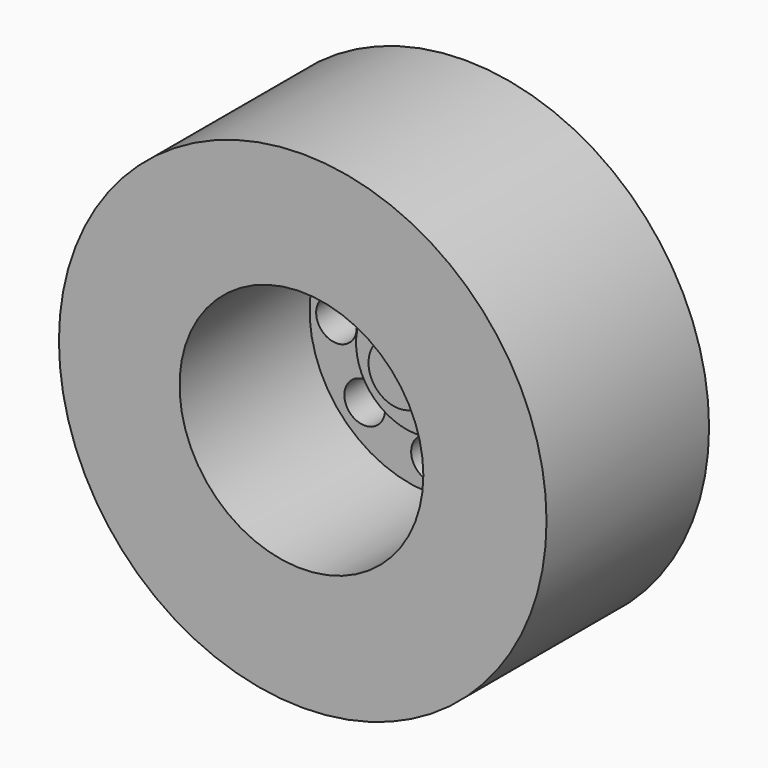
from build123d import *

# Parameters (mm, degrees)
F0_R      = 19.05
F1_DEPTH  = 15.875
F2_R      = 9.525
F3_DEPTH  = 12.7
F4_R      = 1.5875
F5_DEPTH  = 25.4
F6_R      = 1.5875
F7_DEPTH  = 25.4
F8_R      = 1.5875
F9_DEPTH  = 25.4
F10_R     = 1.5875
F11_DEPTH = 25.4
F12_R     = 1.5875
F13_DEPTH = 25.4
F14_R     = 1.5875
F15_DEPTH = 25.4
F16_R     = 1.5875
F17_DEPTH = 25.4
F18_R     = 1.5875
F19_DEPTH = 25.4
F20_R     = 4.7625
F21_DEPTH = 1.5875
F22_R     = 2.38125
F23_DEPTH = 1.5875
F24_R     = 3.175
F25_DEPTH = 9.652
F26_R     = 1.5875
F27_DEPTH = 10.668


# Not quite as in the source:
# - a length typed as a fraction of an inch, garbled in the dataset ("3 / 203.2 mm" for 3/8 in), is restored


with BuildPart() as f1:
    # F0 (on Front) → F1 (new body)
    with BuildSketch(Plane.XZ):
        with Locations((0.1005562392, -0.0107518102)):
            Circle(F0_R)
    extrude(amount=F1_DEPTH)

    # F2 (on face) → F3 (cut)
    with BuildSketch(Plane.XZ.offset(15.875)):
        Circle(F2_R)
    extrude(amount=-F3_DEPTH, mode=Mode.SUBTRACT)

    # F4 (on face) → F5 (cut)
    with BuildSketch(Plane.XZ.offset(3.175)):
        with Locations((0, 7.3800315149)):
            Circle(F4_R)
    extrude(amount=-F5_DEPTH, mode=Mode.SUBTRACT)

    # F6 (on face) → F7 (cut)
    with BuildSketch(Plane.XZ.offset(3.175)):
        with Locations((0, -7.154897321)):
            Circle(F6_R)
    extrude(amount=-F7_DEPTH, mode=Mode.SUBTRACT)

    # F8 (on face) → F9 (cut)
    with BuildSketch(Plane.XZ.offset(3.175)):
        with Locations((7.3278159834, 0)):
            Circle(F8_R)
    extrude(amount=-F9_DEPTH, mode=Mode.SUBTRACT)

    # F10 (on face) → F11 (cut)
    with BuildSketch(Plane.XZ.offset(3.175)):
        with Locations((-7.4240518734, 0)):
            Circle(F10_R)
    extrude(amount=-F11_DEPTH, mode=Mode.SUBTRACT)

    # F12 (on face) → F13 (cut)
    with BuildSketch(Plane.XZ.offset(3.175)):
        with Locations((-5.2546598017, 5.1744827069)):
            Circle(F12_R)
    extrude(amount=-F13_DEPTH, mode=Mode.SUBTRACT)

    # F14 (on face) → F15 (cut)
    with BuildSketch(Plane.XZ.offset(3.175)):
        with Locations((5.3030503914, 4.8490739428)):
            Circle(F14_R)
    extrude(amount=-F15_DEPTH, mode=Mode.SUBTRACT)

    # F16 (on face) → F17 (cut)
    with BuildSketch(Plane.XZ.offset(3.175)):
        with Locations((-5.2185030654, -4.949348513)):
            Circle(F16_R)
    extrude(amount=-F17_DEPTH, mode=Mode.SUBTRACT)

    # F18 (on face) → F19 (cut)
    with BuildSketch(Plane.XZ.offset(3.175)):
        with Locations((5.3030503914, -4.9131917767)):
            Circle(F18_R)
    extrude(amount=-F19_DEPTH, mode=Mode.SUBTRACT)

    # F20 (on face) → F21 (join)
    with BuildSketch(Plane.XZ.offset(3.175)):
        with Locations((0.1396279233, 0.0120795696)):
            Circle(F20_R)
    extrude(amount=F21_DEPTH)

    # F22 (on face) → F23 (join)
    with BuildSketch(Plane.XZ.offset(4.7625)):
        Circle(F22_R)
    extrude(amount=F23_DEPTH)

    # F24 (on face) → F25 (join)
    with BuildSketch(Plane(origin=(0, 0, 0), x_dir=(-1, 0, 0), z_dir=(0, 1, 0))):
        Circle(F24_R)
    extrude(amount=F25_DEPTH)

    # F26 (on face) → F27 (cut)
    with BuildSketch(Plane(origin=(0, 9.652, 0), x_dir=(-1, 0, 0), z_dir=(0, 1, 0))):
        Circle(F26_R)
    extrude(amount=-F27_DEPTH, mode=Mode.SUBTRACT)


solid = f1.part
